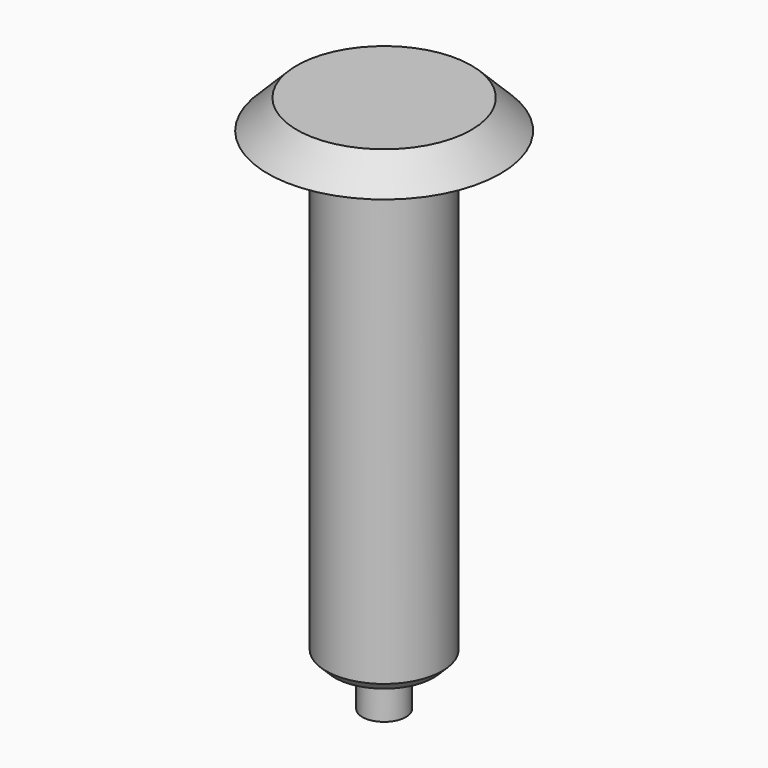
from build123d import *

# Parameters (mm, degrees)
F0_R     = 40
F1_DEPTH = 10
F2_R     = 30
F3_DEPTH = 10
F4_R     = 20
F5_DEPTH = 150
F6_R     = 7.5
F7_DEPTH = 15
F8_SIZE2 = 9.99999
F8_SIZE  = 9.99999
F9_SIZE  = 9.99999
F10_SIZE = 3


# Not quite as in the source:
# - a fillet or chamfer is up to 0.001 mm smaller than in the source, because OpenCascade refuses the exact size


with BuildPart() as f1:
    # F0 (on Top) → F1 (new body)
    with BuildSketch(Plane.XY):
        Circle(F0_R)
    extrude(amount=F1_DEPTH)

    # F2 (on Top) → F3 (join)
    with BuildSketch(Plane.XY):
        Circle(F2_R)
    extrude(amount=-F3_DEPTH)

    # F4 (on face) → F5 (join)
    with BuildSketch(Plane(origin=(0, 0, -10), x_dir=(1, 0, 0), z_dir=(0, 0, -1))):
        Circle(F4_R)
    extrude(amount=F5_DEPTH)

    # F6 (on face) → F7 (join)
    with BuildSketch(Plane(origin=(0, 0, -160), x_dir=(1, 0, 0), z_dir=(0, 0, -1))):
        Circle(F6_R)
    extrude(amount=F7_DEPTH)

    # F8 (size 10 and 10 in the source; OpenCascade refuses exactly that, so slightly less here)
    f8_edges = [f1.edges().sort_by_distance(p)[0] for p in [
        (-40, 0, 10),
    ]]
    chamfer(f8_edges, length=F8_SIZE, length2=F8_SIZE2)

    # F9 (size 10 in the source; OpenCascade refuses exactly that, so slightly less here)
    f9_edges = [f1.edges().sort_by_distance(p)[0] for p in [
        (-30, 0, -10),
    ]]
    chamfer(f9_edges, length=F9_SIZE)

    # F10
    f10_edges = [f1.edges().sort_by_distance(p)[0] for p in [
        (-20, 0, -160),
    ]]
    chamfer(f10_edges, length=F10_SIZE)


solid = f1.part
